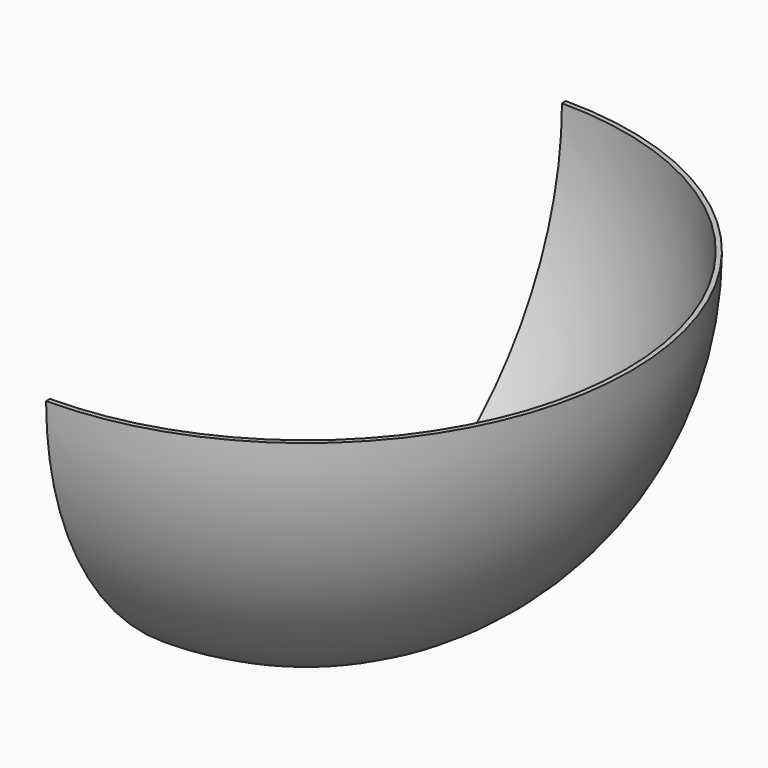
from build123d import *

# Parameters (mm, degrees)
F1_ANGLE_BACK = 90
F1_ANGLE      = 180


with BuildPart() as f1:
    # F0 (on Front) → F1 (revolve)
    with BuildSketch(Plane.XZ, mode=Mode.PRIVATE) as f1_sk:
        with BuildLine():
            ThreePointArc((332, 0), (234.7594513539, -234.7594513539), (0, -332))
            Line((0, -332), (0, -337))
            ThreePointArc((0, -337), (238.2949852599, -238.2949852599), (337, 0))
            Line((337, 0), (332, 0))
        make_face()
    revolve(f1_sk.sketch.rotate(Axis((0, 0, -166), (0, 0, -1)), -F1_ANGLE_BACK), axis=Axis((0, 0, -166), (0, 0, -1)), revolution_arc=F1_ANGLE)


solid = f1.part
